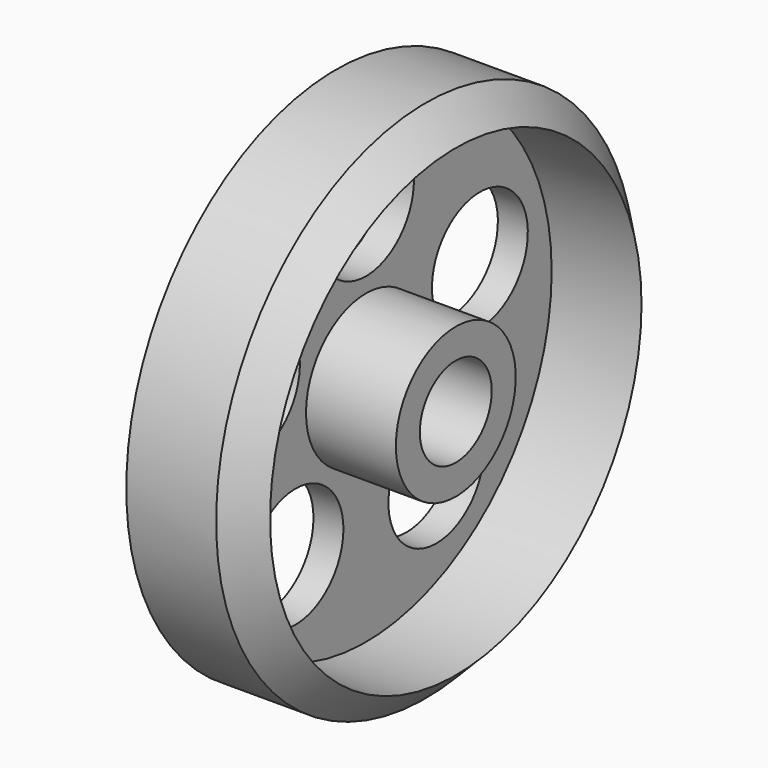
from build123d import *

# Parameters (mm, degrees)
F0_W            = 8
F0_H            = 17.5
F3_D            = 6
F3_DEPTH        = 12
F3_TIP          = 1.8025818571
F4_T            = -2
F6_D            = 8
F6_DEPTH        = 12
F6_TIP          = 2.4034424761
F6_COPIES_COUNT = 5
F7_SIZE         = 1.99999


# Not quite as in the source:
# - a fillet or chamfer is up to 0.001 mm smaller than in the source, because OpenCascade refuses the exact size
# - a pattern or mirror of a feature is missing from the dataset's text; its kind, count and spacing are read off the source's solid


with BuildPart() as f1:
    # F0 (on Top) → F1 (revolve)
    with BuildSketch(Plane.XY):
        with Locations((4, 8.75)):
            Rectangle(F0_W, F0_H)
    revolve(axis=Axis((4, 0, 0), (1, 0, 0)))

    # F3
    with Locations(Plane(origin=(0, 0, 0), x_dir=(0, 1, 0), z_dir=(-1, 0, 0))):
        with Locations((0, 0)):
            Hole(F3_D / 2, depth=F3_DEPTH)
            with Locations((0, 0, -(F3_DEPTH + F3_TIP / 2))):  # 118° drill point
                Cone(0, F3_D / 2, F3_TIP, mode=Mode.SUBTRACT)

    # F4
    f4_openings = [f1.faces().sort_by_distance(p)[0] for p in [
        (8, -17.005025, 0),
    ]]
    offset(amount=F4_T, openings=f4_openings)

    # F6
    with Locations(Plane(origin=(0, 0, 0), x_dir=(0, 1, 0), z_dir=(-1, 0, 0))):
        with Locations((0, -10)):
            f6 = Hole(F6_D / 2, depth=F6_DEPTH)
            with Locations((0, 0, -(F6_DEPTH + F6_TIP / 2))):  # 118° drill point
                Cone(0, F6_D / 2, F6_TIP, mode=Mode.SUBTRACT)

    # F6_copies: F6 ×5 about axis
    f6_copies_axis = Axis((0, 0, 0), (1, 0, 0))
    for i in range(1, F6_COPIES_COUNT):
        add(f6.rotate(f6_copies_axis, i * 360 / F6_COPIES_COUNT), mode=Mode.SUBTRACT)

    # F7 (size 2 in the source; OpenCascade refuses exactly that, so slightly less here)
    f7_edges = [f1.edges().sort_by_distance(p)[0] for p in [
        (8, -17.5, 0),
    ]]
    chamfer(f7_edges, length=F7_SIZE)


solid = f1.part
